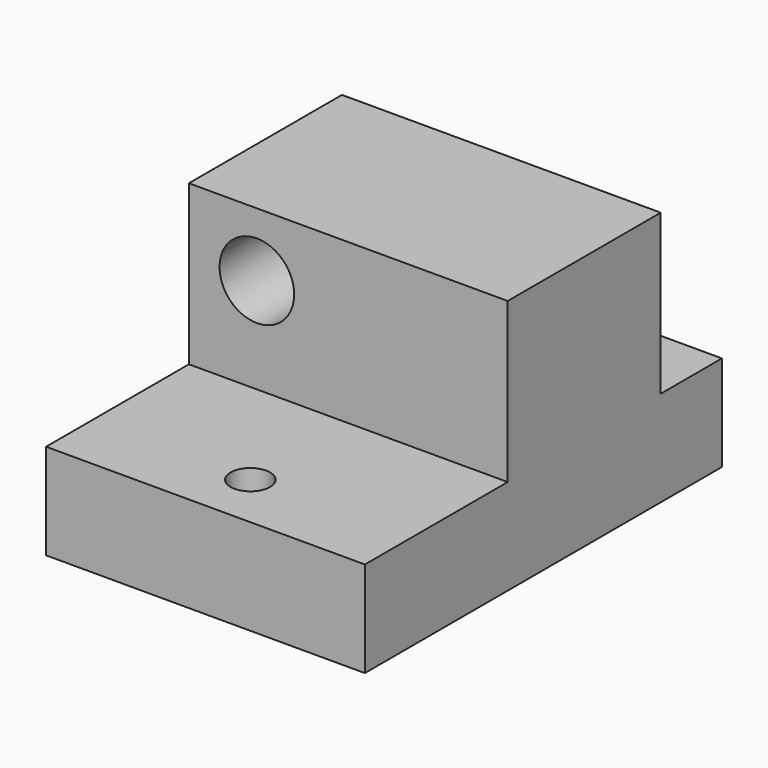
from build123d import *

# Parameters (mm, degrees)
F0_W      = 63.5
F0_H      = 15.24
F0_R      = 3.937
F0_H_2    = 38.1
F0_R_2    = 7.4295
F0_H_3    = 35.56
F1_DEPTH  = 19.05
F5_DEPTH  = 50.8
F7_DEPTH  = 3.175
F2_R      = 11.3792
F9_DEPTH  = 3.175
F6_R      = 7.4295
F10_DEPTH = 19.05
F11_DEPTH = 73.661
F8_R      = 5.08
F12_DEPTH = 31.75


# Not quite as in the source:
# - a feature names something its author has since deleted; it is built from what else it names


with BuildPart() as f1:
    # F0 (on Top) → F1 (new body)
    with BuildSketch(Plane.XY):
        with Locations((31.75, 81.28)):
            Rectangle(F0_W, F0_H)
        with Locations((11.43, 81.28)):
            Circle(F0_R, mode=Mode.SUBTRACT)
        with Locations((52.07, 81.28)):
            Circle(F0_R, mode=Mode.SUBTRACT)
        with Locations((31.75, 54.61)):
            Rectangle(F0_W, F0_H_2)
        with Locations((13.5382, 59.944)):
            Circle(F0_R_2, mode=Mode.SUBTRACT)
        with Locations((49.9618, 59.944)):
            Circle(F0_R_2, mode=Mode.SUBTRACT)
        with Locations((13.5382, 59.944)):
            Circle(F0_R_2)
        with Locations((49.9618, 59.944)):
            Circle(F0_R_2)
        with Locations((31.75, 17.78)):
            Rectangle(F0_W, F0_H_3)
        with Locations((31.75, 11.176)):
            Circle(F0_R, mode=Mode.SUBTRACT)
    extrude(amount=F1_DEPTH)


with BuildPart() as f3_1:
    # F3: copy of F1
    add(f1.part.moved(Location((-152.4, 0, 0))))


with BuildPart() as f1_1:
    add(f1.part)

    # F0 (on Top) → F5 (join)
    with BuildSketch(Plane.XY):
        with Locations((31.75, 54.61)):
            Rectangle(F0_W, F0_H_2)
        with Locations((13.5382, 59.944)):
            Circle(F0_R_2, mode=Mode.SUBTRACT)
        with Locations((49.9618, 59.944)):
            Circle(F0_R_2, mode=Mode.SUBTRACT)
        with Locations((49.9618, 59.944)):
            Circle(F0_R_2)
        with Locations((13.5382, 59.944)):
            Circle(F0_R_2)
    extrude(amount=F5_DEPTH)

    # F0 (on Top) → F7 (cut)
    with BuildSketch(Plane.XY):
        with Locations((49.9618, 59.944)):
            Circle(F0_R_2)
        with Locations((13.5382, 59.944)):
            Circle(F0_R_2)
    extrude(amount=F7_DEPTH, mode=Mode.SUBTRACT)

    # F2 (on face) → F9 (cut)
    with BuildSketch(Plane(origin=(0, 0, 0), x_dir=(1, 0, 0), z_dir=(0, 0, -1))):
        with Locations((49.9618, -59.944)):
            Circle(F2_R)
        with Locations((13.5382, -59.944)):
            Circle(F2_R)
    extrude(amount=-F9_DEPTH, mode=Mode.SUBTRACT)

    # F6 (on face) → F10 (cut)
    with BuildSketch(Plane(origin=(0, 73.66, 0), x_dir=(-1, 0, 0), z_dir=(0, 1, 0))):
        with Locations((-49.9618, 38.1)):
            Circle(F6_R)
    extrude(amount=-F10_DEPTH, mode=Mode.SUBTRACT)

    # F6 (on face) → F11 (cut, through all)
    with BuildSketch(Plane(origin=(0, 73.66, 0), x_dir=(-1, 0, 0), z_dir=(0, 1, 0))):
        with Locations((-13.5382, 38.1)):
            Circle(F6_R)
    extrude(amount=-F11_DEPTH, mode=Mode.SUBTRACT)

    # F8 (on face) → F12 (cut)
    with BuildSketch(Plane(origin=(0, 0, 3.175), x_dir=(1, 0, 0), z_dir=(0, 0, -1))):
        with Locations((49.9618, -59.944)):
            Circle(F8_R)
    extrude(amount=-F12_DEPTH, mode=Mode.SUBTRACT)


solid = f1_1.part
